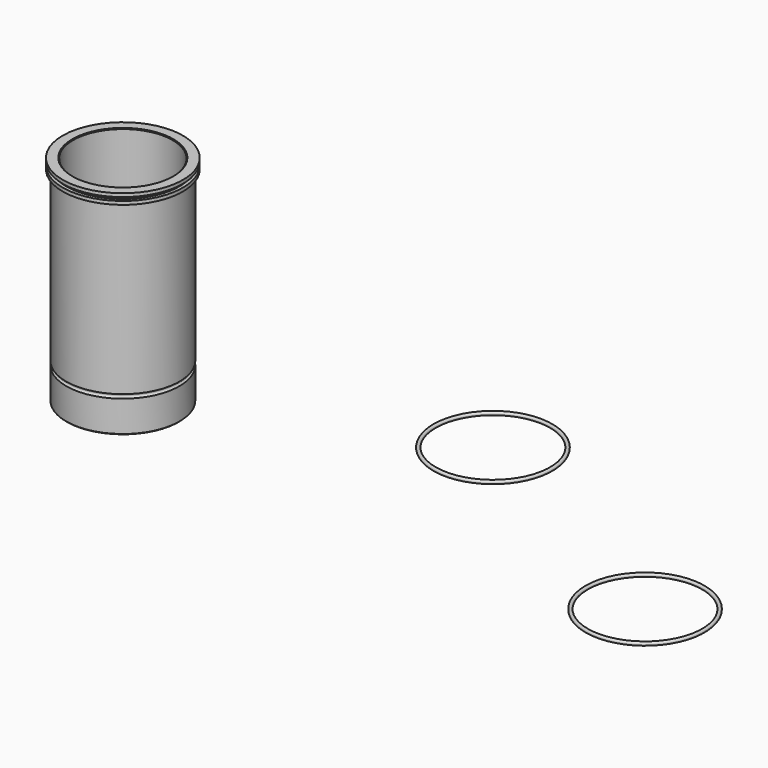
from build123d import *

# Parameters (mm, degrees)
F3_R = 1
F6_R = 1


# Not quite as in the source:
# - a fillet or chamfer that OpenCascade refuses, or shapes differently, is made with other operations: its cross-section is extruded or revolved along the edge and cut away or added


with BuildPart() as f1:
    # F0 (on Front) → F1 (revolve)
    with BuildSketch(Plane.XZ):
        with BuildLine():
            Line((-29, 125), (-35, 125))
            Line((-35, 125), (-35, 123))
            Line((-35, 123), (-33, 123))
            Line((-33, 123), (-33, 121))
            Line((-33, 121), (-35, 121))
            Line((-35, 121), (-35, 119))
            Line((-35, 119), (-33, 119))
            Line((-33, 119), (-33, 20.5190867633))
            ThreePointArc((-33, 20.5190867633), (-32.0398381638, 19.5190867633), (-33, 18.5190867633))
            Line((-33, 18.5190867633), (-33, 0))
            Line((-33, 0), (-29, 0))
            Line((-29, 0), (-29, 125))
        make_face()
    revolve(axis=Axis((0, 0, 70.6444829702), (0, 0, 1)))

    # F2: chamfer of 0.4 on 5 edges, made by hand

    # F2_s1 → F2_t2 (revolve)
    with BuildSketch(Plane.XZ):
        Polygon((-33.4, 119), (-33, 118.6), (-33, 119), align=None)
    revolve(axis=Axis((0, 0, 119), (0, 0, 1)))

    # F2_s3 → F2_t4 (revolve, cut)
    with BuildSketch(Plane.XZ):
        Polygon((-29.4, 125), (-29, 124.6), (-29, 125), align=None)
    revolve(axis=Axis((0, 0, 125), (0, 0, 1)), mode=Mode.SUBTRACT)

    # F2_s5 → F2_t6 (revolve, cut)
    with BuildSketch(Plane.XZ):
        Polygon((-29, 0.4), (-29.4, 0), (-29, 0), align=None)
    revolve(axis=Axis((0, 0, 0), (0, 0, 1)), mode=Mode.SUBTRACT)

    # F2_s7 → F2_t8 (revolve, cut)
    with BuildSketch(Plane.XZ):
        with BuildLine():
            Line((-32.7258298981, 20.4691039761), (-33, 20.8487970584))
            Line((-33, 20.8487970584), (-33, 20.5190867633))
            ThreePointArc((-33, 20.5190867633), (-32.8554047109, 20.5026173296), (-32.7258298981, 20.4691039761))
        make_face()
    revolve(axis=Axis((0, 0, 20.5190867633), (0, 0, 1)), mode=Mode.SUBTRACT)

    # F2_s9 → F2_t10 (revolve, cut)
    with BuildSketch(Plane.XZ):
        Polygon((-32.6, 0), (-33, 0.4), (-33, 0), align=None)
    revolve(axis=Axis((0, 0, 0), (0, 0, 1)), mode=Mode.SUBTRACT)


with BuildPart() as f4:
    # F3 (on Front) → F4 (revolve)
    with BuildSketch(Plane.XZ):
        with Locations((270.3552097399, -7.6474512478)):
            Circle(F3_R)
    revolve(axis=Axis((304.3552097399, 0, 1.5939064324), (0, 0, -1)))


with BuildPart() as f4b:
    # F3 (on Front) → F4, piece 2 (revolve)
    with BuildSketch(Plane.XZ):
        with Locations((185.3699033564, 49.2150506932)):
            Circle(F3_R)
    revolve(axis=Axis((304.3552097399, 0, 1.5939064324), (0, 0, -1)))


with BuildPart() as f7:
    # F6 (on Front) → F7 (revolve)
    with BuildSketch(Plane.XZ):
        with Locations((181.7116728007, 46.4359594094)):
            Circle(F6_R)
    revolve(axis=Axis((215.7116728007, 0, 69.0873954445), (0, 0, -1)))


solid = Compound([f1.part, f4.part, f7.part])
